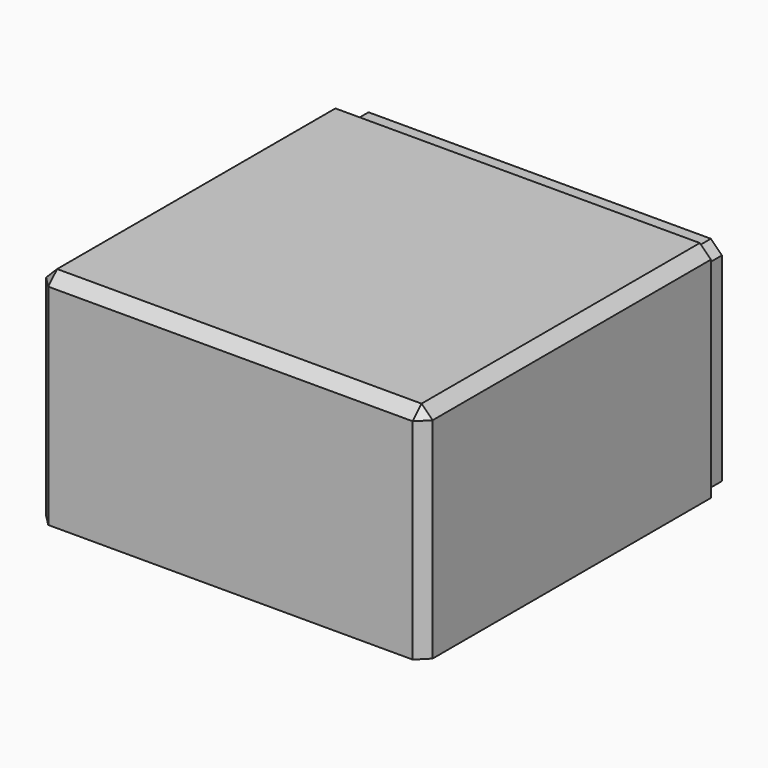
from build123d import *

# Parameters (mm, degrees)
F0_R        = 1.45
F0_W        = 66
F0_H        = 5
F1_DEPTH    = 40
F2_DEPTH    = 38
F3_SIZE     = 2
F4_T        = 2.5
F4_T3_DEPTH = 41
F4_T5_DEPTH = 7.8284271247
F4_T7_DEPTH = 67
F4_T9_DEPTH = 7.8284271247
F5_START    = 20
F5_DEPTH    = 20


# Not quite as in the source:
# - a shell that OpenCascade refuses in one call is made with other operations: the cavity is built on its own and cut out


with BuildPart() as f1:
    # F0 (on Top) → F1 (new body)
    with BuildSketch(Plane.XY):
        Polygon((-33, 32.5), (-35, 32.5), (-35, -32.5), (35, -32.5), (35, 32.5), (33, 32.5), (33, 27.5), (-33, 27.5), align=None)
        with Locations((-30, -27.5)):
            Circle(F0_R, mode=Mode.SUBTRACT)
        with Locations((30, -27.5)):
            Circle(F0_R, mode=Mode.SUBTRACT)
        with Locations((0, 30)):
            Rectangle(F0_W, F0_H)
    extrude(amount=F1_DEPTH)

    # F0 (on Top) → F2 (join)
    with BuildSketch(Plane.XY):
        Polygon((-33, 32.5), (-35, 32.5), (-35, -32.5), (35, -32.5), (35, 32.5), (33, 32.5), (33, 27.5), (-33, 27.5), align=None)
        with Locations((-30, -27.5)):
            Circle(F0_R, mode=Mode.SUBTRACT)
        with Locations((30, -27.5)):
            Circle(F0_R, mode=Mode.SUBTRACT)
        with Locations((0, 35)):
            Rectangle(F0_W, F0_H)
        with Locations((0, 30)):
            Rectangle(F0_W, F0_H)
    extrude(amount=F2_DEPTH)

    # F3
    f3_edges = [f1.edges().sort_by_distance(p)[0] for p in [
        (0, -32.5, 40),
        (35, 0, 40),
        (-35, 0, 40),
        (33, 35, 38),
        (-33, 35, 38),
        (-35, -32.5, 20),
        (35, -32.5, 20),
    ]]
    chamfer(f3_edges, length=F3_SIZE)

    # F4: shell of thickness 2.5, made by hand


with BuildPart() as f4_core1:
    # F4_t2: copy of F1
    add(f1.part)

    # the walls: a layer under each face that stays
    f4_faces = [f4_core1.faces().sort_by_distance(p)[0] for p in [
        (-35, 1, 19),
        (-34, -31.5, 19),
        (32.6666666667, 32.5, 38.6666666667),
        (-34, 1, 39),
        (0, -32.5, 19),
        (-33, 35, 18),
        (34, -31.5, 19),
        (35, 1, 19),
        (33, 35, 18),
        (-31.45, -27.5, 20),
        (28.55, -27.5, 20),
        (-34, -31, 38.5),
        (-32, 35, 37),
        (0, 35, 38),
        (32, 35, 37),
        (0, 1, 40),
        (34, 1, 39),
        (0, -31.5, 39),
        (34, -31, 38.5),
    ]]
    thicken(f4_faces, amount=-F4_T, mode=Mode.SUBTRACT)

    # F4_s4 → F4_t3 (cut)
    with BuildSketch(Plane.XY.offset(-2.5)):
        Polygon((-33.025, 32.525), (-33, 30), (-30.5, 30), (-30.5, 32.5), align=None)
        Polygon((33.025, 32.525), (33, 30), (30.5, 30), (30.5, 32.5), align=None)
    extrude(amount=F4_T3_DEPTH, mode=Mode.SUBTRACT)

    # F4_s6 → F4_t5 (cut)
    with BuildSketch(Plane(origin=(5.267766953, 0, 5.267766953), x_dir=(0, 1, 0), z_dir=(-0.7071067812, 0, -0.7071067812))):
        Polygon((32.525, -48.8153679019), (30, -48.7903679019), (30, -46.2903679019), (32.5, -46.2903679019), align=None)
    extrude(amount=F4_T5_DEPTH, mode=Mode.SUBTRACT)

    # F4_s8 → F4_t7 (cut)
    with BuildSketch(Plane.YZ.offset(-33.5)):
        Polygon((32.525, 38.025), (30, 38), (30, 35.5), (32.5, 35.5), align=None)
    extrude(amount=F4_T7_DEPTH, mode=Mode.SUBTRACT)

    # F4_s10 → F4_t9 (cut)
    with BuildSketch(Plane(origin=(0.267766953, 0, -0.267766953), x_dir=(0, 1, 0), z_dir=(-0.7071067812, 0, 0.7071067812))):
        Polygon((32.525, -48.8153679019), (30, -48.7903679019), (30, -46.2903679019), (32.5, -46.2903679019), align=None)
    extrude(amount=F4_T9_DEPTH, mode=Mode.SUBTRACT)


with BuildPart() as f1_1:
    add(f1.part)

    # what is left inside the walls is the cavity
    f4_cavity = [f4_core1.part.solids().sort_by_distance(p)[0] for p in [
        (0, -7.5, 0.025),
    ]]
    add(f4_cavity, mode=Mode.SUBTRACT)

    # F0 (on Top) → F5 (join)
    with BuildSketch(Plane.XY.offset(F5_START)):
        with Locations((-30, -27.5)):
            Circle(F0_R)
        with Locations((30, -27.5)):
            Circle(F0_R)
    extrude(amount=F5_DEPTH)


solid = f1_1.part
